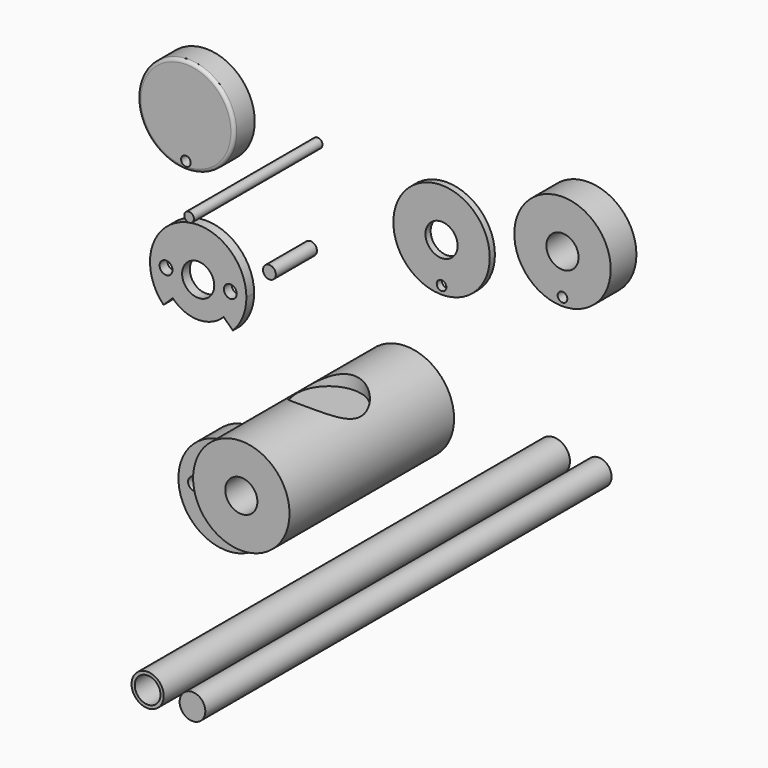
from build123d import *

# Parameters (mm, degrees)
F0_R      = 15
F0_R_2    = 5
F1_DEPTH  = 64
F2_R      = 2
F2_R_2    = 5
F3_DEPTH  = 3
F4_R      = 15
F4_R_2    = 2
F4_R_3    = 5
F5_DEPTH  = 10
F6_R      = 15
F6_R_2    = 1.5
F6_R_3    = 5
F7_DEPTH  = 2
F9_R      = 10
F10_DEPTH = 4
F11_R     = 5
F11_R_2   = 4
F12_DEPTH = 158
F13_R     = 4
F14_DEPTH = 158
F15_R     = 2
F16_DEPTH = 16
F17_R     = 15
F17_R_2   = 1.5
F18_DEPTH = 8
F19_R     = 1.5
F20_DEPTH = 50
F21_R     = 0.99999
F17_R_3   = 5
F22_DEPTH = 10
F23_R     = 5
F24_DEPTH = 5


# Not quite as in the source:
# - a fillet or chamfer is up to 0.001 mm smaller than in the source, because OpenCascade refuses the exact size
# - a feature names something its author has since deleted; it is built from what else it names


with BuildPart() as f1:
    # F0 (on Front) → F1 (new body)
    with BuildSketch(Plane.XZ):
        Circle(F0_R)
        Circle(F0_R_2, mode=Mode.SUBTRACT)
    extrude(amount=F1_DEPTH)

    # F9 (on offset) → F10 (cut)
    with BuildSketch(Plane.XY.offset(15)):
        with Locations((0, -30)):
            Circle(F9_R)
    extrude(amount=-F10_DEPTH, mode=Mode.SUBTRACT)


with BuildPart() as f3:
    # F2 (on Front) → F3 (new body)
    with BuildSketch(Plane.XZ):
        with BuildLine():
            Line((-54.3058665821, 6.5412230759), (-51.4285073808, 3.7625895941))
            ThreePointArc((-51.4285073808, 3.7625895941), (-48.3108465674, 8.5633662497), (-47.2186043859, 14.182465151))
            ThreePointArc((-47.2186043859, 14.182465151), (-67.8377032871, 28.0902229695), (-73.0087013909, 3.7625895941))
            Line((-73.0087013909, 3.7625895941), (-70.1313421896, 6.5412230759))
            ThreePointArc((-70.1313421896, 6.5412230759), (-62.2186043859, 3.182465151), (-54.3058665821, 6.5412230759))
        make_face()
        with Locations((-72.2186043859, 14.182465151)):
            Circle(F2_R, mode=Mode.SUBTRACT)
        with Locations((-62.2186043859, 14.182465151)):
            Circle(F2_R_2, mode=Mode.SUBTRACT)
        with BuildLine():
            ThreePointArc((-54.2186043859, 14.182465151), (-52.2186043859, 16.182465151), (-50.2186043859, 14.182465151))
            ThreePointArc((-50.2186043859, 14.182465151), (-52.2186043859, 12.182465151), (-54.2186043859, 14.182465151))
        make_face(mode=Mode.SUBTRACT)
    extrude(amount=F3_DEPTH)


with BuildPart() as f5:
    # F4 (on Front) → F5 (new body)
    with BuildSketch(Plane.XZ):
        with Locations((-47.7725118399, -37.5088863075)):
            Circle(F4_R)
        with Locations((-57.7725118399, -37.5088863075)):
            Circle(F4_R_2, mode=Mode.SUBTRACT)
        with Locations((-47.7725118399, -37.5088863075)):
            Circle(F4_R_3, mode=Mode.SUBTRACT)
        with Locations((-37.7725118399, -37.5088863075)):
            Circle(F4_R_2, mode=Mode.SUBTRACT)
    extrude(amount=F5_DEPTH)


with BuildPart() as f7:
    # F6 (on Front) → F7 (new body)
    with BuildSketch(Plane.XZ):
        with Locations((12.6999374479, 49.0343069208)):
            Circle(F6_R)
        with Locations((12.6999374479, 36.5343069208)):
            Circle(F6_R_2, mode=Mode.SUBTRACT)
        with Locations((12.6999374479, 49.0343069208)):
            Circle(F6_R_3, mode=Mode.SUBTRACT)
    extrude(amount=F7_DEPTH)


with BuildPart() as f12:
    # F11 (on Front) → F12 (new body)
    with BuildSketch(Plane.XZ):
        with Locations((46.0497015125, 0)):
            Circle(F11_R)
        with Locations((46.0497015125, 0)):
            Circle(F11_R_2, mode=Mode.SUBTRACT)
    extrude(amount=F12_DEPTH)


with BuildPart() as f14:
    # F13 (on Front) → F14 (new body)
    with BuildSketch(Plane.XZ):
        with Locations((60, 0)):
            Circle(F13_R)
    extrude(amount=F14_DEPTH)


with BuildPart() as f16:
    # F15 (on Front) → F16 (new body)
    with BuildSketch(Plane.XZ):
        with Locations((-29.6608433127, 32.0971570909)):
            Circle(F15_R)
    extrude(amount=F16_DEPTH)


with BuildPart() as f18:
    # F17 (on Front) → F18 (new body)
    with BuildSketch(Plane.XZ):
        with Locations((-62.032982707, 61.2359903753)):
            Circle(F17_R)
        with Locations((-62.032982707, 48.7359903753)):
            Circle(F17_R_2, mode=Mode.SUBTRACT)
    extrude(amount=F18_DEPTH)

    # F21 (radius 1 in the source; OpenCascade refuses exactly that, so slightly less here)
    f21_edges = [f18.edges().sort_by_distance(p)[0] for p in [
        (-77.032983, -8, 61.23599),
    ]]
    fillet(f21_edges, radius=F21_R)

    # F23 (on face) → F24 (cut)
    with BuildSketch(Plane(origin=(0, 0, 0), x_dir=(-1, 0, 0), z_dir=(0, 1, 0))):
        with Locations((62.032982707, 61.2359903753)):
            Circle(F23_R)
    extrude(amount=-F24_DEPTH, mode=Mode.SUBTRACT)


with BuildPart() as f20:
    # F19 (on Front) → F20 (new body)
    with BuildSketch(Plane.XZ):
        with Locations((-27.4534914643, 61.705391854)):
            Circle(F19_R)
    extrude(amount=F20_DEPTH)


with BuildPart() as f22:
    # F17 (on Front) → F22 (new body)
    with BuildSketch(Plane.XZ):
        with Locations((56.7282065749, 63.4172449509)):
            Circle(F17_R)
        with Locations((56.7282065749, 50.9172449509)):
            Circle(F17_R_2, mode=Mode.SUBTRACT)
        with Locations((56.7282065749, 63.4172449509)):
            Circle(F17_R_3, mode=Mode.SUBTRACT)
    extrude(amount=F22_DEPTH)


solid = Compound([f1.part, f3.part, f5.part, f7.part, f12.part, f14.part, f16.part, f18.part, f20.part, f22.part])
